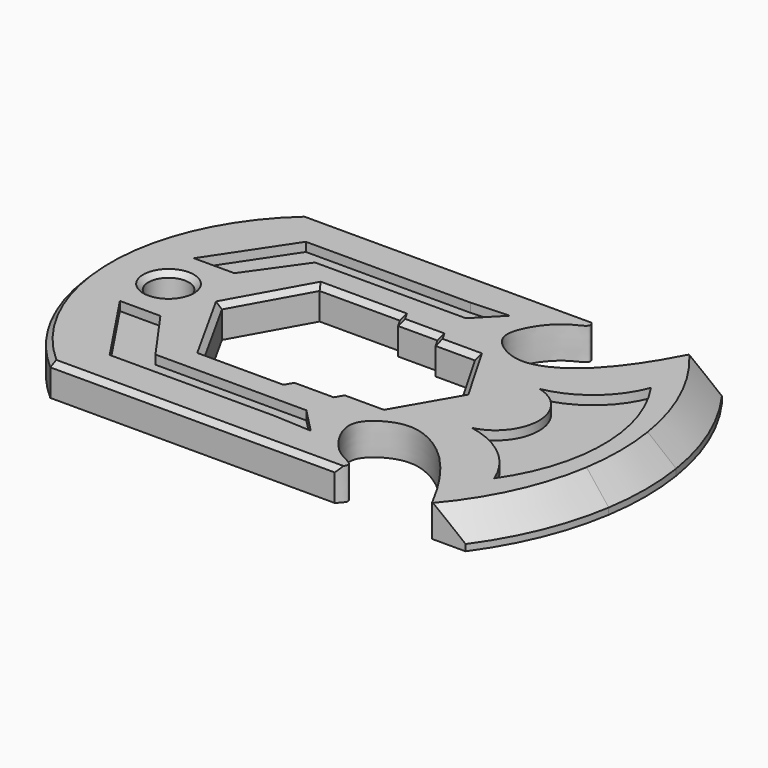
from build123d import *

# Parameters (mm, degrees)
F0_R     = 2
F1_DEPTH = 3.175
F2_SIZE2 = 2.54
F2_SIZE  = 2.54
F3_SIZE  = 0.508
F4_DEPTH = 2.286
F5_DEPTH = 2.286


# Not quite as in the source:
# - a feature names something its author has since deleted; it is built from what else it names


with BuildPart() as f1:
    # F0 (on Top) → F1 (new body)
    with BuildSketch(Plane.XY):
        with BuildLine():
            Line((-25.4, -9.7533396771), (-25.4, 9.7533396771))
            ThreePointArc((-25.4, 9.7533396771), (-27.7943947705, 0), (-25.4, -9.7533396771))
        make_face()
        with BuildLine():
            Line((7.5996425003, 15.875), (-20.574, 15.875))
            ThreePointArc((-20.574, 15.875), (-23.2726776835, 13.0393833309), (-25.4, 9.7533396771))
            Line((-25.4, 9.7533396771), (-25.4, -9.7533396771))
            ThreePointArc((-25.4, -9.7533396771), (-23.2726776835, -13.0393833309), (-20.574, -15.875))
            Line((-20.574, -15.875), (7.5996425003, -15.875))
            add(Edge.make_bspline(
                [(17.2575954348, -15.875), (16.8118674755, -15.0360308318), (15.7777378861, -13.0895457095), (12.6385533239, -8.7628284751), (8.4438454096, -6.4903546022), (5.4576611574, -7.5578133093), (3.6996913649, -9.434816458), (4.9096520026, -12.30721807), (6.6995754798, -14.1477736043), (8.6865320781, -14.7997007485), (7.9445844593, -15.5337364181), (7.5996425003, -15.875)],
                knots=[0, 0, 0, 0, 0.1172509784, 0.2720329825, 0.4136469471, 0.5269156212, 0.6254604471, 0.7364742974, 0.8471369559, 0.9289318052, 1, 1, 1, 1], degree=3))
            Line((17.2575954348, -15.875), (19.5524021983, -15.875))
            ThreePointArc((19.5524021983, -15.875), (24.535980368, 0), (19.5524021983, 15.875))
            Line((19.5524021983, 15.875), (17.2575954348, 15.875))
            add(Edge.make_bspline(
                [(17.2575954348, 15.875), (16.8118674755, 15.0360308318), (15.7777378861, 13.0895457095), (12.6385533239, 8.7628284751), (8.4438454096, 6.4903546022), (5.4576611574, 7.5578133093), (3.6996913649, 9.434816458), (4.9096520026, 12.30721807), (6.6995754798, 14.1477736043), (8.6865320781, 14.7997007485), (7.9445844593, 15.5337364181), (7.5996425003, 15.875)],
                knots=[0, 0, 0, 0, 0.1172509784, 0.2720329825, 0.4136469471, 0.5269156212, 0.6254604471, 0.7364742974, 0.8471369559, 0.9289318052, 1, 1, 1, 1], degree=3))
        make_face()
        Polygon((0, -9.8765036091), (2.4003, -12.3413112015), (-1.3600544771, -12.1478205547), (-17.6725629717, -12.1478205547), (-22.7162260562, -4.5817312784), (-18.6995025724, -4.5817312784), (-14.9566456676, -9.8765036091), align=None, mode=Mode.SUBTRACT)
        with Locations((-21.5576495975, 0)):
            Circle(F0_R, mode=Mode.SUBTRACT)
        Polygon((-16.2712801248, 0), (-12.2982449182, 7.1374), (-4.3480449182, 7.1374), (-3.8934393163, 6.35), (0, 6.35), (0.4617137668, 5.5502882974), (4.3540745974, 5.5502882974), (7.5559447504, 0.0061843585), (4.3434, -5.5581063708), (0.4572, -5.5581063708), (0, -6.35), (-3.8934393163, -6.35), (-4.3480449182, -7.1374), (-12.2982449182, -7.1374), align=None, mode=Mode.SUBTRACT)
        Polygon((-14.9566456676, 9.8765036091), (-18.6995025724, 4.5817312784), (-22.7162260562, 4.5817312784), (-17.6725629717, 12.1478205547), (-1.3600544771, 12.1478205547), (2.4003, 12.3413112015), (0, 9.8765036091), align=None, mode=Mode.SUBTRACT)
        with BuildLine():
            ThreePointArc((18.4671971947, -9.7006708384), (15.8776249613, -6.080528756), (11.8529647589, -4.1796281002))
            ThreePointArc((11.8529647589, -4.1796281002), (15.1365712278, 0.0061843585), (11.8529647589, 4.1919968173))
            ThreePointArc((11.8529647589, 4.1919968173), (15.8776249613, 6.092897473), (18.4671971947, 9.7130395554))
            ThreePointArc((18.4671971947, 9.7130395554), (21.5143278197, 0.0061843585), (18.4671971947, -9.7006708384))
        make_face(mode=Mode.SUBTRACT)
        with BuildLine():
            ThreePointArc((25.4, -4.1788812389), (25.7248773783, 0), (25.4, 4.1788812389))
            Line((25.4, 4.1788812389), (25.4, -4.1788812389))
        make_face()
        with BuildLine():
            Line((20.574, 15.875), (19.5524021983, 15.875))
            ThreePointArc((19.5524021983, 15.875), (24.535980368, 0), (19.5524021983, -15.875))
            Line((19.5524021983, -15.875), (20.574, -15.875))
            ThreePointArc((20.574, -15.875), (23.6807693851, -10.3132006276), (25.4, -4.1788812389))
            Line((25.4, -4.1788812389), (25.4, 4.1788812389))
            ThreePointArc((25.4, 4.1788812389), (23.6807693851, 10.3132006276), (20.574, 15.875))
        make_face()
    extrude(amount=F1_DEPTH)

    # F2
    f2_edges = [f1.edges().sort_by_distance(p)[0] for p in [
        (25.724877, 0, 3.175),
    ]]
    chamfer(f2_edges, length=F2_SIZE, length2=F2_SIZE2)

    # F3
    f3_edges = [f1.edges().sort_by_distance(p)[0] for p in [
        (-23.55765, 0, 3.175),
        (-14.284763, 3.5687, 3.175),
        (-14.284763, -3.5687, 3.175),
        (-8.323145, -7.1374, 3.175),
        (-8.323145, 7.1374, 3.175),
        (-4.120742, -6.7437, 3.175),
        (-1.94672, -6.35, 3.175),
        (0.2286, -5.954053, 3.175),
        (2.4003, -5.558106, 3.175),
        (5.949672, -2.775961, 3.175),
        (5.95501, 2.778236, 3.175),
        (-4.120742, 6.7437, 3.175),
        (-1.94672, 6.35, 3.175),
        (0.230857, 5.950144, 3.175),
        (2.407894, 5.550288, 3.175),
        (-6.487179, 15.875, 3.175),
        (-27.794395, 0, 3.175),
        (-6.487179, -15.875, 3.175),
    ]]
    chamfer(f3_edges, length=F3_SIZE)

    # F0 (on Top) → F4 (join)
    with BuildSketch(Plane.XY):
        Polygon((-1.3600544771, -12.1478205547), (2.4003, -12.3413112015), (0, -9.8765036091), (-14.9566456676, -9.8765036091), (-18.6995025724, -4.5817312784), (-22.7162260562, -4.5817312784), (-17.6725629717, -12.1478205547), align=None)
        Polygon((-22.7162260562, 4.5817312784), (-18.6995025724, 4.5817312784), (-14.9566456676, 9.8765036091), (0, 9.8765036091), (2.4003, 12.3413112015), (-1.3600544771, 12.1478205547), (-17.6725629717, 12.1478205547), align=None)
    extrude(amount=F4_DEPTH)

    # F0 (on Top) → F5 (join)
    with BuildSketch(Plane.XY):
        with BuildLine():
            ThreePointArc((11.8529647589, 4.1919968173), (15.1365712278, 0.0061843585), (11.8529647589, -4.1796281002))
            ThreePointArc((11.8529647589, -4.1796281002), (15.8776249613, -6.080528756), (18.4671971947, -9.7006708384))
            ThreePointArc((18.4671971947, -9.7006708384), (21.5143278197, 0.0061843585), (18.4671971947, 9.7130395554))
            ThreePointArc((18.4671971947, 9.7130395554), (15.8776249613, 6.092897473), (11.8529647589, 4.1919968173))
        make_face()
    extrude(amount=F5_DEPTH)


solid = f1.part
